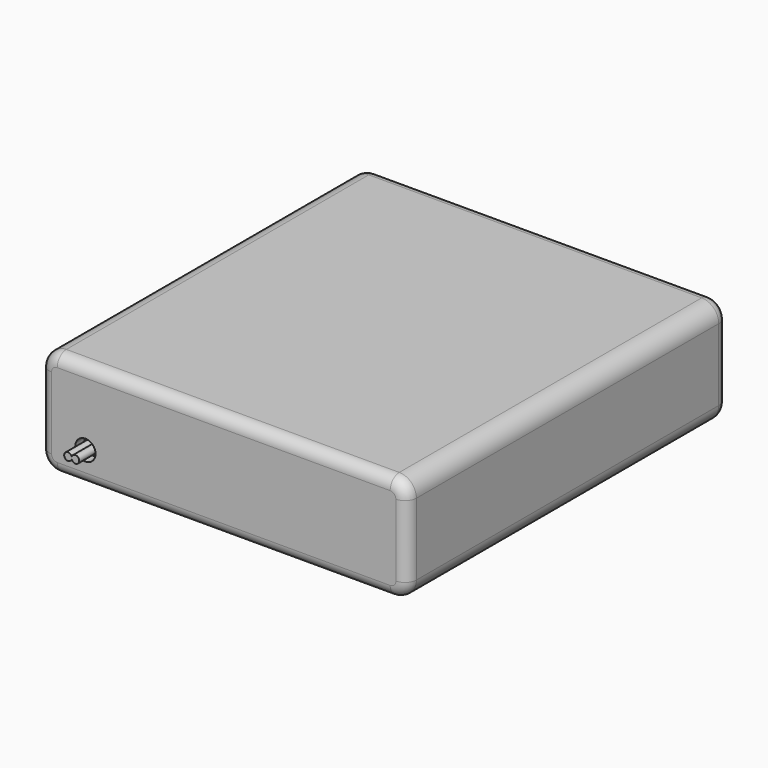
from build123d import *

# Parameters (mm, degrees)
F0_W          = 64.45
F0_H          = 70.35
F1_DEPTH      = 18.65
F2_R          = 3
F3_R          = 2
F4_W          = 8.2
F4_H          = 4.35
F5_DEPTH      = 2.5
F6_W          = 3
F6_H          = 3
F7_DEPTH      = 3.8
F8_R          = 1.78
F9_DEPTH      = 2
F10_TEXT_SIZE = 3.2406108841
F11_DEPTH     = 0.5
F14_ANGLE     = 180
F16_ANGLE     = 90
F18_ANGLE     = 90
F20_DEPTH     = 5


# Not quite as in the source:
# - Text() gives the source's letters only with a copy of the font that has no kerning and outlines rounded to 1/6400 em; it was checked with that copy


with BuildPart() as f1:
    # F0 (on Top) → F1 (new body)
    with BuildSketch(Plane.XY):
        Rectangle(F0_W, F0_H)
    extrude(amount=F1_DEPTH)

    # F2
    f2_edges = [f1.edges().sort_by_distance(p)[0] for p in [
        (-32.225, 0, 18.65),
        (32.225, 0, 18.65),
        (32.225, 0, 0),
        (-32.225, 0, 0),
    ]]
    fillet(f2_edges, radius=F2_R)

    # F3
    f3_edges = [f1.edges().sort_by_distance(p)[0] for p in [
        (-32.225, -35.175, 9.325),
        (-31.34632, -35.175, 0.87868),
        (-31.34632, -35.175, 17.77132),
        (0, -35.175, 0),
        (0, -35.175, 18.65),
        (31.34632, -35.175, 0.87868),
        (31.34632, -35.175, 17.77132),
        (32.225, -35.175, 9.325),
        (32.225, 35.175, 9.325),
        (31.34632, 35.175, 0.87868),
        (31.34632, 35.175, 17.77132),
        (0, 35.175, 0),
        (0, 35.175, 18.65),
        (-31.34632, 35.175, 0.87868),
        (-31.34632, 35.175, 17.77132),
        (-32.225, 35.175, 9.325),
    ]]
    fillet(f3_edges, radius=F3_R)

    # F4 (on face) → F5 (cut)
    with BuildSketch(Plane.XY.offset(18.65)):
        with Locations((20.625, 29.4)):
            Rectangle(F4_W, F4_H)
    extrude(amount=-F5_DEPTH, mode=Mode.SUBTRACT)

    # F6 (on face) → F7 (join)
    with BuildSketch(Plane.XY.offset(16.15)):
        with Locations((18.7, 29.4)):
            Rectangle(F6_W, F6_H)
    extrude(amount=F7_DEPTH)

    # F8 (on face) → F9 (cut)
    with BuildSketch(Plane(origin=(0, 35.175, 0), x_dir=(-1, 0, 0), z_dir=(0, 1, 0))):
        with Locations((24.285, 13.14)):
            Circle(F8_R)
    extrude(amount=-F9_DEPTH, mode=Mode.SUBTRACT)

    # F10 (on face) → F11 (join)
    with BuildSketch(Plane.XY.offset(18.65)):
        with Locations((14.74, 23.3917601635)):
            Text('OFF-ON', F10_TEXT_SIZE, font='Open Sans', text_align=(TextAlign.LEFT, TextAlign.BOTTOM))
    extrude(amount=F11_DEPTH)


with BuildPart() as f1_1:
    # F14: moved
    add(f1.part.rotate(Axis((0, 0.7596462965, 0), (0, -1, 0)), F14_ANGLE))


with BuildPart() as f1_2:
    # F16: moved
    add(f1_1.part.rotate(Axis((0, 0, 19.4975901395), (0, 0, 1)), F16_ANGLE))


with BuildPart() as f1_3:
    # F18: moved
    add(f1_2.part.rotate(Axis((0, 0, 29.9103371799), (0, 0, 1)), F18_ANGLE))

    # F19 (on face) → F20 (join)
    with BuildSketch(Plane.XZ.offset(33.175)):
        with BuildLine():
            ThreePointArc((-24.285, -13.3220027472), (-22.96, -13.14), (-24.285, -12.9579972528))
            ThreePointArc((-24.285, -12.9579972528), (-25.61, -13.14), (-24.285, -13.3220027472))
        make_face()
    extrude(amount=F20_DEPTH)


solid = f1_3.part
